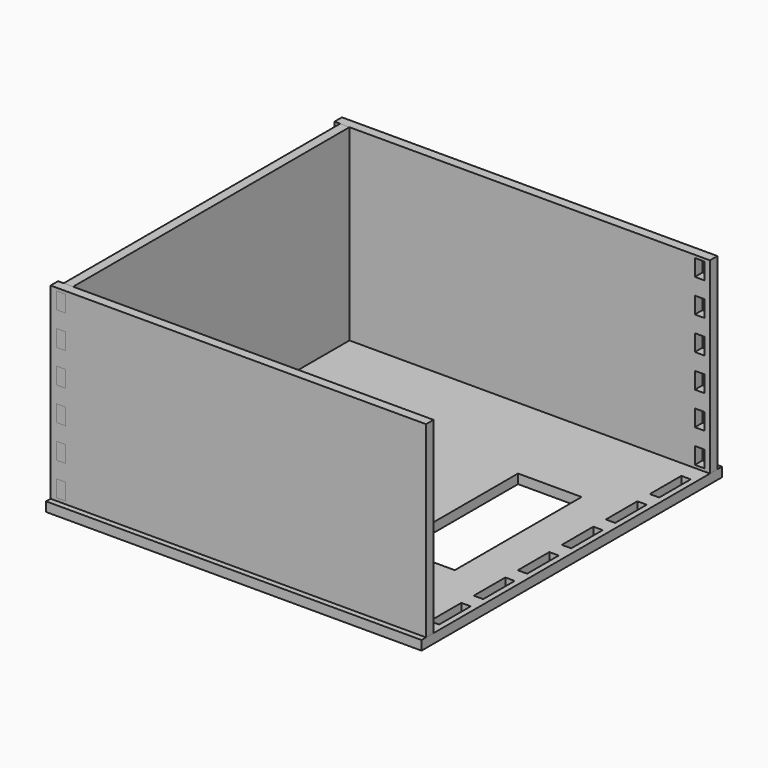
from build123d import *

# Parameters (mm, degrees)
F1_W      = 200
F1_H      = 200
F2_DEPTH  = 5
F3_W      = 20
F3_H      = 5
F4_DEPTH  = 25
F5_W      = 20
F5_H      = 5
F6_DEPTH  = 5
F7_W      = 200
F7_H      = 5
F8_DEPTH  = 100
F9_W      = 5
F9_H      = 21
F10_DEPTH = 25
F12_W     = 5
F12_H     = 10
F13_DEPTH = 25
F14_W     = 5
F14_H     = 184
F15_DEPTH = 100
F16_DEPTH = 5
F19_W     = 5
F19_H     = 8.8473876119
F20_DEPTH = 25
F21_DEPTH = 5
F23_W     = 5
F23_H     = 8.8473876119
F24_DEPTH = 25
F25_W     = 5
F25_H     = 8.847
F26_DEPTH = 25
F27_DEPTH = 5
F28_W     = 33.871
F28_H     = 84.4354853034
F29_DEPTH = 25


with BuildPart() as f2:
    # F1 (on Top) → F2 (new body)
    with BuildSketch(Plane.XY):
        Rectangle(F1_W, F1_H)
    extrude(amount=F2_DEPTH)

    # F3 (on face) → F4 (cut)
    with BuildSketch(Plane.XY.offset(5)):
        with Locations((-87, 94.5)):
            Rectangle(F3_W, F3_H)
        with Locations((-52.2, 94.5)):
            Rectangle(F3_W, F3_H)
        with Locations((-17.4, 94.5)):
            Rectangle(F3_W, F3_H)
        with Locations((17.4, 94.5)):
            Rectangle(F3_W, F3_H)
        with Locations((52.2, 94.5)):
            Rectangle(F3_W, F3_H)
        with Locations((87, 94.5)):
            Rectangle(F3_W, F3_H)
        with Locations((-87, -94.5)):
            Rectangle(F3_W, F3_H)
        with Locations((87, -94.5)):
            Rectangle(F3_W, F3_H)
        with Locations((-52.2, -94.5)):
            Rectangle(F3_W, F3_H)
        with Locations((52.2, -94.5)):
            Rectangle(F3_W, F3_H)
        with Locations((-17.4, -94.5)):
            Rectangle(F3_W, F3_H)
        with Locations((17.4, -94.5)):
            Rectangle(F3_W, F3_H)
    extrude(amount=-F4_DEPTH, mode=Mode.SUBTRACT)

    # F9 (on face) → F10 (cut)
    with BuildSketch(Plane(origin=(0, 0, 0), x_dir=(1, 0, 0), z_dir=(0, 0, -1))):
        with Locations((94.5, 74.025)):
            Rectangle(F9_W, F9_H)
        with Locations((94.5, 44.72)):
            Rectangle(F9_W, F9_H)
        with Locations((94.5, 15.415)):
            Rectangle(F9_W, F9_H)
        with Locations((94.5, -13.89)):
            Rectangle(F9_W, F9_H)
        with Locations((94.5, -43.195)):
            Rectangle(F9_W, F9_H)
        with Locations((94.5, -72.5)):
            Rectangle(F9_W, F9_H)
        with Locations((-94.5, 74.025)):
            Rectangle(F9_W, F9_H)
        with Locations((-94.5, 44.72)):
            Rectangle(F9_W, F9_H)
        with Locations((-94.5, 15.415)):
            Rectangle(F9_W, F9_H)
        with Locations((-94.5, -13.89)):
            Rectangle(F9_W, F9_H)
        with Locations((-94.5, -43.195)):
            Rectangle(F9_W, F9_H)
        with Locations((-94.5, -72.5)):
            Rectangle(F9_W, F9_H)
    extrude(amount=-F10_DEPTH, mode=Mode.SUBTRACT)

    # F12 (on face) → F13 (cut)
    with BuildSketch(Plane.XZ.offset(-92)):
        with Locations((-144.5, 97)):
            Rectangle(F12_W, F12_H)
        with Locations((-144.5, 80.2)):
            Rectangle(F12_W, F12_H)
        with Locations((-144.5, 63.4)):
            Rectangle(F12_W, F12_H)
        with Locations((-144.5, 46.6)):
            Rectangle(F12_W, F12_H)
        with Locations((-144.5, 29.8)):
            Rectangle(F12_W, F12_H)
        with Locations((-144.5, 13)):
            Rectangle(F12_W, F12_H)
        with Locations((144.5, 97)):
            Rectangle(F12_W, F12_H)
        with Locations((144.5, 80.2)):
            Rectangle(F12_W, F12_H)
        with Locations((144.5, 63.4)):
            Rectangle(F12_W, F12_H)
        with Locations((144.5, 46.6)):
            Rectangle(F12_W, F12_H)
        with Locations((144.5, 29.8)):
            Rectangle(F12_W, F12_H)
        with Locations((144.5, 13)):
            Rectangle(F12_W, F12_H)
    extrude(amount=-F13_DEPTH, mode=Mode.SUBTRACT)

    # F28 (on face) → F29 (cut)
    with BuildSketch(Plane.XY.offset(5)):
        with Locations((-54.5564480126, 0)):
            Rectangle(F28_W, F28_H)
        with Locations((54.5564480126, 0)):
            Rectangle(F28_W, F28_H)
    extrude(amount=-F29_DEPTH, mode=Mode.SUBTRACT)


with BuildPart() as f6:
    # F5 (on face) → F6 (new body, through all)
    with BuildSketch(Plane.XY.offset(5)):
        with Locations((-52.2, 94.5)):
            Rectangle(F5_W, F5_H)
    extrude(amount=-F6_DEPTH)



with BuildPart() as f6b:
    # F5 (on face) → F6, piece 2 (new body, through all)
    with BuildSketch(Plane.XY.offset(5)):
        with Locations((-87, 94.5)):
            Rectangle(F5_W, F5_H)
    extrude(amount=-F6_DEPTH)


with BuildPart() as f6c:
    # F5 (on face) → F6, piece 3 (new body, through all)
    with BuildSketch(Plane.XY.offset(5)):
        with Locations((-17.4, 94.5)):
            Rectangle(F5_W, F5_H)
    extrude(amount=-F6_DEPTH)


with BuildPart() as f6d:
    # F5 (on face) → F6, piece 4 (new body, through all)
    with BuildSketch(Plane.XY.offset(5)):
        with Locations((17.4, 94.5)):
            Rectangle(F5_W, F5_H)
    extrude(amount=-F6_DEPTH)


with BuildPart() as f6e:
    # F5 (on face) → F6, piece 5 (new body, through all)
    with BuildSketch(Plane.XY.offset(5)):
        with Locations((52.2, 94.5)):
            Rectangle(F5_W, F5_H)
    extrude(amount=-F6_DEPTH)


with BuildPart() as f6f:
    # F5 (on face) → F6, piece 6 (new body, through all)
    with BuildSketch(Plane.XY.offset(5)):
        with Locations((87, 94.5)):
            Rectangle(F5_W, F5_H)
    extrude(amount=-F6_DEPTH)


with BuildPart() as f6_1:
    add(f6.part)

    add(f6b.part)  # F8 merges F6b

    add(f6c.part)  # F8 merges F6c

    add(f6d.part)  # F8 merges F6d

    add(f6e.part)  # F8 merges F6e

    add(f6f.part)  # F8 merges F6f
    # F7 (on face) → F8 (join)
    with BuildSketch(Plane.XY.offset(5)):
        with Locations((0, 94.5)):
            Rectangle(F7_W, F7_H)
    extrude(amount=F8_DEPTH)

    # F11: union 


with BuildPart() as f15:
    # F14 (on face) → F15 (new body)
    with BuildSketch(Plane.XY.offset(5)):
        with Locations((-94.5, 0)):
            Rectangle(F14_W, F14_H)
    extrude(amount=F15_DEPTH)

    # F9 (on face) → F16 (join, through all)
    with BuildSketch(Plane(origin=(0, 0, 0), x_dir=(1, 0, 0), z_dir=(0, 0, -1))):
        with Locations((-94.5, 74.025)):
            Rectangle(F9_W, F9_H)
        with Locations((-94.5, 44.72)):
            Rectangle(F9_W, F9_H)
        with Locations((-94.5, 15.415)):
            Rectangle(F9_W, F9_H)
        with Locations((-94.5, -13.89)):
            Rectangle(F9_W, F9_H)
        with Locations((-94.5, -43.195)):
            Rectangle(F9_W, F9_H)
        with Locations((-94.5, -72.5)):
            Rectangle(F9_W, F9_H)
    extrude(amount=-F16_DEPTH)

    # F17: union 

    # F19 (on face) → F21 (join, through all)
    with BuildSketch(Plane.XZ.offset(-92)):
        with Locations((-94.5, 99.0763061941)):
            Rectangle(F19_W, F19_H)
        with Locations((-94.5, 81.4457837164)):
            Rectangle(F19_W, F19_H)
        with Locations((-94.5, 63.8152612388)):
            Rectangle(F19_W, F19_H)
        with Locations((-94.5, 46.1847387612)):
            Rectangle(F19_W, F19_H)
        with Locations((-94.5, 28.5542162836)):
            Rectangle(F19_W, F19_H)
        with Locations((-94.5, 10.9236938059)):
            Rectangle(F19_W, F19_H)
    extrude(amount=-F21_DEPTH)

    # F22: union 

    # F25 (on face) → F27 (join, through all)
    with BuildSketch(Plane(origin=(0, -92, 0), x_dir=(-1, 0, 0), z_dir=(0, 1, 0))):
        with Locations((94.45, 99.0785)):
            Rectangle(F25_W, F25_H)
        with Locations((94.45, 81.4475)):
            Rectangle(F25_W, F25_H)
        with Locations((94.45, 63.8165)):
            Rectangle(F25_W, F25_H)
        with Locations((94.45, 46.1855)):
            Rectangle(F25_W, F25_H)
        with Locations((94.45, 28.5545)):
            Rectangle(F25_W, F25_H)
        with Locations((94.45, 10.9235)):
            Rectangle(F25_W, F25_H)
    extrude(amount=-F27_DEPTH)


with BuildPart() as f18_1:
    # F18: copy of F6
    add(f6_1.part.moved(Location((0, -189, 0))))

    # F25 (on face) → F26 (cut)
    with BuildSketch(Plane(origin=(0, -92, 0), x_dir=(-1, 0, 0), z_dir=(0, 1, 0))):
        with Locations((94.45, 99.0785)):
            Rectangle(F25_W, F25_H)
        with Locations((94.45, 81.4475)):
            Rectangle(F25_W, F25_H)
        with Locations((94.45, 63.8165)):
            Rectangle(F25_W, F25_H)
        with Locations((94.45, 46.1855)):
            Rectangle(F25_W, F25_H)
        with Locations((94.45, 28.5545)):
            Rectangle(F25_W, F25_H)
        with Locations((94.45, 10.9235)):
            Rectangle(F25_W, F25_H)
    extrude(amount=-F26_DEPTH, mode=Mode.SUBTRACT)


with BuildPart() as f6_2:
    add(f6_1.part)

    # F19 (on face) → F20 (cut)
    with BuildSketch(Plane.XZ.offset(-92)):
        with Locations((-94.5, 99.0763061941)):
            Rectangle(F19_W, F19_H)
        with Locations((-94.5, 81.4457837164)):
            Rectangle(F19_W, F19_H)
        with Locations((-94.5, 63.8152612388)):
            Rectangle(F19_W, F19_H)
        with Locations((-94.5, 46.1847387612)):
            Rectangle(F19_W, F19_H)
        with Locations((-94.5, 28.5542162836)):
            Rectangle(F19_W, F19_H)
        with Locations((-94.5, 10.9236938059)):
            Rectangle(F19_W, F19_H)
    extrude(amount=-F20_DEPTH, mode=Mode.SUBTRACT)

    # F23 (on face) → F24 (cut)
    with BuildSketch(Plane.XZ.offset(-92)):
        with Locations((94.5, 99.0763061941)):
            Rectangle(F23_W, F23_H)
        with Locations((94.5, 81.4457837164)):
            Rectangle(F23_W, F23_H)
        with Locations((94.5, 28.5542162836)):
            Rectangle(F23_W, F23_H)
        with Locations((94.5, 63.8152612388)):
            Rectangle(F23_W, F23_H)
        with Locations((94.5, 10.9236938059)):
            Rectangle(F23_W, F23_H)
        with Locations((94.5, 46.1847387612)):
            Rectangle(F23_W, F23_H)
    extrude(amount=-F24_DEPTH, mode=Mode.SUBTRACT)


solid = Compound([f2.part, f15.part, f18_1.part, f6_2.part])
